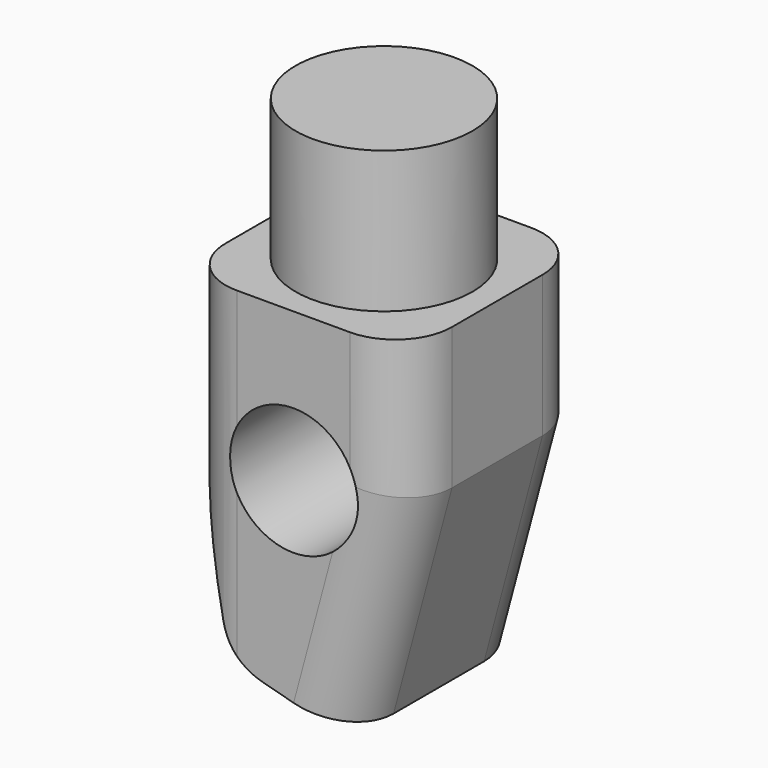
from build123d import *

# Parameters (mm, degrees)
F0_W        = 20.32
F0_H        = 38.1
F1_DEPTH    = 20.32
F2_SIZE2    = 6.8059094878
F2_SIZE     = 25.4
F2_2_SIZE2  = 6.8059094878
F2_2_SIZE   = 25.4
F3_R        = 5.715
F4_DEPTH    = 25.4
F5_W        = 68.5800006613
F5_H        = 10.5876065791
F6_DEPTH    = 35.56
F7_R        = 7.9375
F8_DEPTH    = 12.7
F9_T1_DEPTH = 46.99
F9_T3_DEPTH = 54.5211276147
F9_T5_DEPTH = 34.9846968374
F9_T7_DEPTH = 23.6639734387


# Not quite as in the source:
# - a fillet or chamfer that OpenCascade refuses, or shapes differently, is made with other operations: its cross-section is extruded or revolved along the edge and cut away or added


with BuildPart() as f1:
    # F0 (on Right) → F1 (new body)
    with BuildSketch(Plane.YZ):
        with Locations((-27.8230281547, -4.4044164286)):
            Rectangle(F0_W, F0_H)
    extrude(amount=F1_DEPTH)

    # F2
    f2_edges = [f1.edges().sort_by_distance(p)[0] for p in [
        (20.32, -27.823028, -23.454416),
    ]]
    f2_side = f1.faces().sort_by_distance((20.32, -27.823028, -4.404416))[0]
    chamfer(f2_edges, length=F2_SIZE, length2=F2_SIZE2, reference=f2_side)

    # F2#2
    f2_2_edges = [f1.edges().sort_by_distance(p)[0] for p in [
        (0, -27.823028, -23.454416),
    ]]
    f2_2_side = f1.faces().sort_by_distance((0, -27.823028, -4.404416))[0]
    chamfer(f2_2_edges, length=F2_2_SIZE, length2=F2_2_SIZE2, reference=f2_2_side)

    # F3 (on face) → F4 (cut)
    with BuildSketch(Plane.XZ.offset(37.9830281547)):
        with Locations((10.16, 1.2867113903)):
            Circle(F3_R)
    extrude(amount=-F4_DEPTH, mode=Mode.SUBTRACT)

    # F5 (on face) → F6 (cut)
    with BuildSketch(Plane(origin=(18.4724222096, 0, -4.9496706133), x_dir=(0, 1, 0), z_dir=(0.9659258263, 0, -0.2588190451))):
        with Locations((-23.6119744368, -18.386438489)):
            Rectangle(F5_W, F5_H)
    extrude(amount=-F6_DEPTH, mode=Mode.SUBTRACT)

    # F7 (on face) → F8 (join)
    with BuildSketch(Plane.XY.offset(14.6455835714)):
        with Locations((10.16, -27.8230281547)):
            Circle(F7_R)
    extrude(amount=F8_DEPTH)

    # F9: fillet of radius 5.08 on 8 edges, made by hand

    # F9_s2 → F9_t1 (cut)
    with BuildSketch(Plane.XY.offset(-19.6444164286)):
        with BuildLine():
            ThreePointArc((20.32, -22.7430281547), (18.8321024484, -19.1509257062), (15.24, -17.6630281547))
            Line((15.24, -17.6630281547), (20.32, -17.6630281547))
            Line((20.32, -17.6630281547), (20.32, -22.7430281547))
        make_face()
        with BuildLine():
            ThreePointArc((0, -22.7430281547), (1.4878975516, -19.1509257062), (5.08, -17.6630281547))
            Line((5.08, -17.6630281547), (0, -17.6630281547))
            Line((0, -17.6630281547), (0, -22.7430281547))
        make_face()
        with BuildLine():
            ThreePointArc((5.08, -37.9830281547), (1.4878975516, -36.4951306031), (0, -32.9030281547))
            Line((0, -32.9030281547), (0, -37.9830281547))
            Line((0, -37.9830281547), (5.08, -37.9830281547))
        make_face()
        with BuildLine():
            ThreePointArc((15.24, -37.9830281547), (18.8321024484, -36.4951306031), (20.32, -32.9030281547))
            Line((20.32, -32.9030281547), (20.32, -37.9830281547))
            Line((20.32, -37.9830281547), (15.24, -37.9830281547))
        make_face()
    extrude(amount=F9_T1_DEPTH, mode=Mode.SUBTRACT)

    # F9_s4 → F9_t3 (cut)
    with BuildSketch(Plane(origin=(7.4354809742, 0, 27.7495927742), x_dir=(0, 1, 0), z_dir=(-0.2588190451, 0, -0.9659258263))):
        with BuildLine():
            ThreePointArc((-37.9830281547, 14.0440587081), (-36.4951306031, 17.6361611565), (-32.9030281547, 19.1240587081))
            Line((-32.9030281547, 19.1240587081), (-37.9830281547, 19.1240587081))
            Line((-37.9830281547, 19.1240587081), (-37.9830281547, 14.0440587081))
        make_face()
        with BuildLine():
            ThreePointArc((-22.7430281547, 19.1240587081), (-19.1509257062, 17.6361611565), (-17.6630281547, 14.0440587081))
            Line((-17.6630281547, 14.0440587081), (-17.6630281547, 19.1240587081))
            Line((-17.6630281547, 19.1240587081), (-22.7430281547, 19.1240587081))
        make_face()
    extrude(amount=F9_T3_DEPTH, mode=Mode.SUBTRACT)

    # F9_s6 → F9_t5 (cut)
    with BuildSketch(Plane.XZ.offset(10.330679736)):
        with BuildLine():
            ThreePointArc((7.3074886766, -15.5125290504), (5.0301869773, -14.1977283012), (3.7153862282, -11.9204266019))
            Line((3.7153862282, -11.9204266019), (4.4744867946, -14.7534284839))
            Line((4.4744867946, -14.7534284839), (7.3074886766, -15.5125290504))
        make_face()
    extrude(amount=F9_T5_DEPTH, mode=Mode.SUBTRACT)

    # F9_s8 → F9_t7 (cut)
    with BuildSketch(Plane.XZ.offset(15.9910414353)):
        with BuildLine():
            ThreePointArc((0, 2.6143782591), (0.0434601042, 1.9513052026), (0.1730968025, 1.29957751))
            Line((0.1730968025, 1.29957751), (0, 1.9455835714))
            Line((0, 1.9455835714), (0, 2.6143782591))
        make_face()
    extrude(amount=F9_T7_DEPTH, mode=Mode.SUBTRACT)


solid = f1.part
